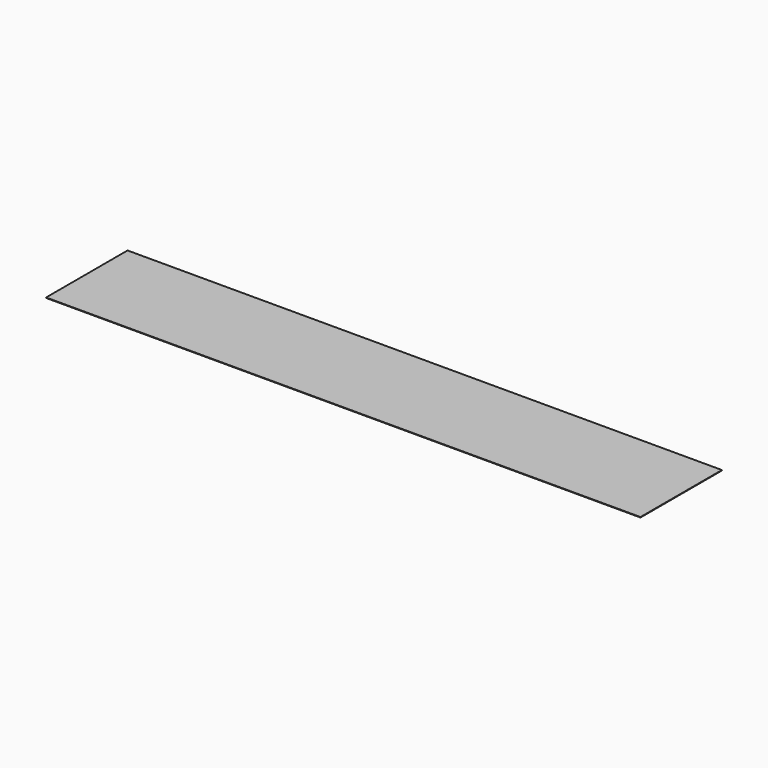
from build123d import *

# Parameters (mm, degrees)
F0_W     = 2048
F0_H     = 350.8
F1_DEPTH = 1.5875


# Not quite as in the source:
# - a length typed as a fraction of an inch, garbled in the dataset ("3 / 203.2 mm" for 3/8 in), is restored


with BuildPart() as f1:
    # F0 (on Top) → F1 (new body)
    with BuildSketch(Plane.XY):
        Rectangle(F0_W, F0_H)
    extrude(amount=F1_DEPTH)


solid = f1.part
